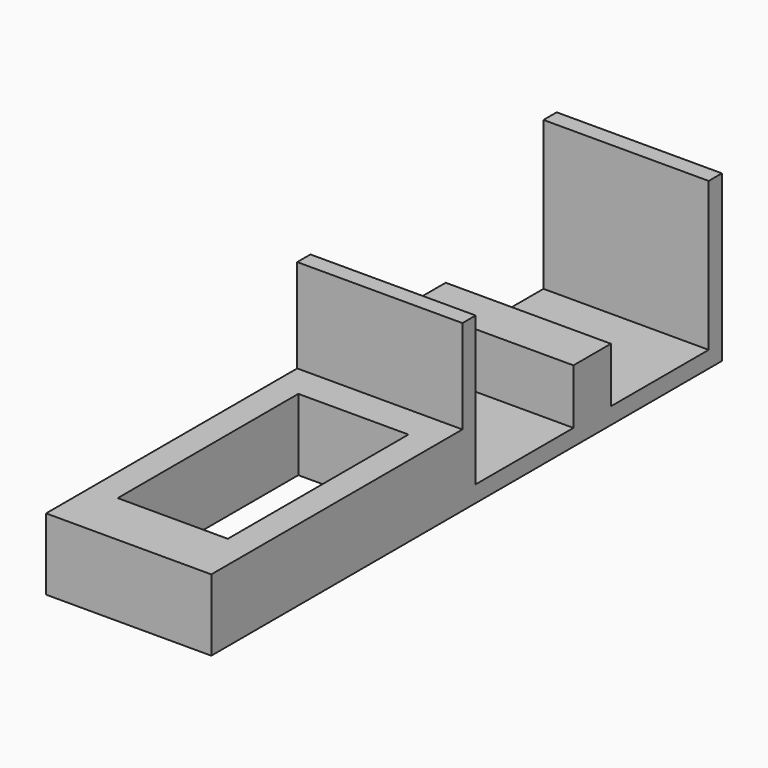
from build123d import *

# Parameters (mm, degrees)
F0_W     = 30
F0_H     = 57
F0_H_2   = 3
F0_H_3   = 22.2
F0_H_4   = 8.5
F1_DEPTH = 3
F2_DEPTH = 30
F3_DEPTH = 13
F4_DEPTH = 10
F5_W     = 20
F5_H     = 41
F6_DEPTH = 13


# Not quite as in the source:
# - a feature of the source that left no trace in its solid (it failed there, or was rolled back) is left out


with BuildPart() as f1:
    # F0 (on Top) → F1 (new body)
    with BuildSketch(Plane.XY):
        with Locations((67.8492219866, 28.5)):
            Rectangle(F0_W, F0_H)
        with Locations((67.8492219866, 58.5)):
            Rectangle(F0_W, F0_H_2)
        with Locations((67.8492219866, 71.1)):
            Rectangle(F0_W, F0_H_3)
        with Locations((67.8492219866, 86.45)):
            Rectangle(F0_W, F0_H_4)
        with Locations((67.8492219866, 101.8)):
            Rectangle(F0_W, F0_H_3)
        with Locations((67.8492219866, 114.4)):
            Rectangle(F0_W, F0_H_2)
    extrude(amount=F1_DEPTH)

    # F0 (on Top) → F2 (join)
    with BuildSketch(Plane.XY):
        with Locations((67.8492219866, 58.5)):
            Rectangle(F0_W, F0_H_2)
        with Locations((67.8492219866, 114.4)):
            Rectangle(F0_W, F0_H_2)
    extrude(amount=F2_DEPTH)

    # F0 (on Top) → F3 (join)
    with BuildSketch(Plane.XY):
        with Locations((67.8492219866, 86.45)):
            Rectangle(F0_W, F0_H_4)
    extrude(amount=F3_DEPTH)

    # F4 (add): a face of the model
    f4_faces = [f1.faces().sort_by_distance(p)[0] for p in [
        (67.8492219866, 28.5, 3),
    ]]
    extrude(f4_faces, amount=F4_DEPTH)

    # F5 (on face) → F6 (cut, through all)
    with BuildSketch(Plane.XY.offset(13)):
        with Locations((67.8492219866, 30.5)):
            Rectangle(F5_W, F5_H)
    extrude(amount=-F6_DEPTH, mode=Mode.SUBTRACT)


solid = f1.part
